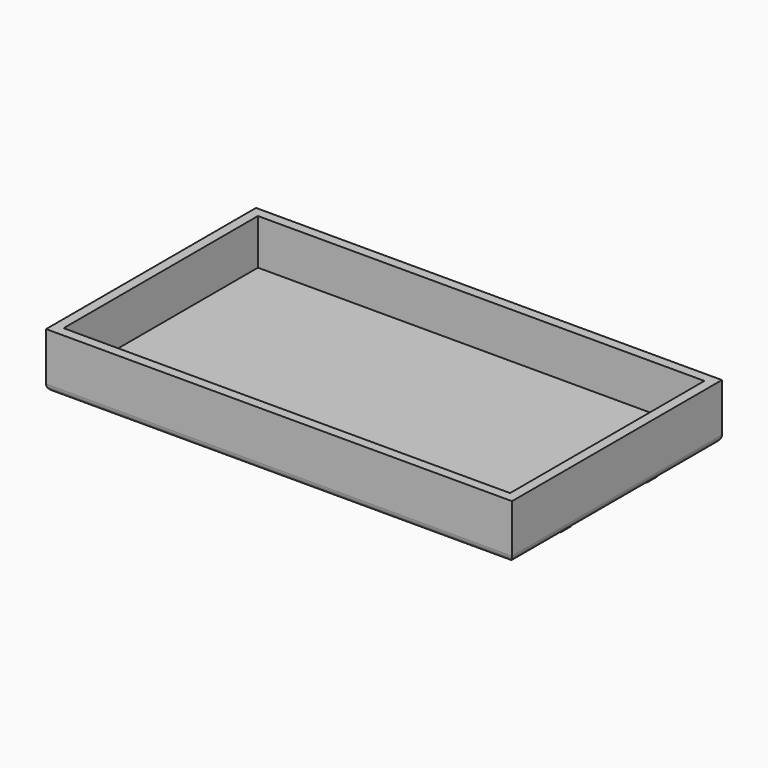
from build123d import *

# Parameters (mm, degrees)
F0_W         = 121.5698868036
F0_H         = 68.4608668089
F1_DEPTH     = 14.4127849489
F2_T         = -2.54
F3_R         = 1.778
F4_TEXT_SIZE = 44.0427357597
F5_DEPTH     = 3.0706878752


# Not quite as in the source:
# - Text() gives the source's letters only with a copy of the font that has no kerning and outlines rounded to 1/6400 em; it was checked with that copy


with BuildPart() as f1:
    # F0 (on Top) → F1 (new body)
    with BuildSketch(Plane.XY):
        with Locations((7.0535168052, 13.484723866)):
            Rectangle(F0_W, F0_H)
    extrude(amount=F1_DEPTH)

    # F2
    f2_openings = [f1.faces().sort_by_distance(p)[0] for p in [
        (7.053517, 13.484724, 14.412785),
    ]]
    offset(amount=F2_T, openings=f2_openings)

    # F3
    f3_edges = [f1.edges().sort_by_distance(p)[0] for p in [
        (7.053517, 47.715157, 0),
        (-53.731427, 13.484724, 0),
        (7.053517, -20.74571, 0),
        (67.83846, 13.484724, 0),
    ]]
    fillet(f3_edges, radius=F3_R)

    # F4 (on face) → F5 (join)
    with BuildSketch(Plane(origin=(0, 0, 0), x_dir=(1, 0, 0), z_dir=(0, 0, -1))):
        with Locations((-51.9534265966, -32.4135384673)):
            Text('HOPE', F4_TEXT_SIZE, font='Open Sans', text_align=(TextAlign.LEFT, TextAlign.BOTTOM))
    extrude(amount=F5_DEPTH)


solid = f1.part
